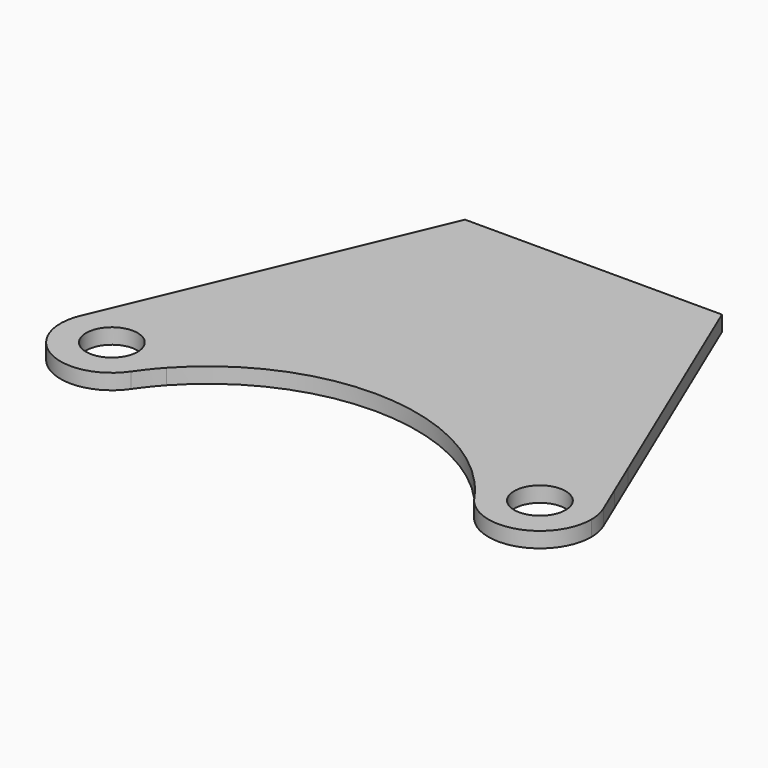
from build123d import *

# Parameters (mm, degrees)
F0_R     = 10
F1_DEPTH = 6


with BuildPart() as f1:
    # F0 (on Top) → F1 (new body)
    with BuildSketch(Plane.XY):
        with BuildLine():
            ThreePointArc((66.8107155763, 68.8983527146), (89.2220086446, 61.1485010982), (103.2801650714, 80.2454771665))
            ThreePointArc((103.2801650714, 80.2454771665), (102.8817929615, 84.2174016446), (101.7025466654, 88.0310957293))
            ThreePointArc((101.7025466654, 88.0310957293), (73.6640874011, 97.7820404055), (66.8107155763, 68.8983527146))
        make_face()
        with Locations((83.2801650714, 80.2454771665)):
            Circle(F0_R, mode=Mode.SUBTRACT)
        with BuildLine():
            ThreePointArc((66.8107155763, 68.8983527146), (73.6640874011, 97.7820404055), (101.7025466654, 88.0310957293))
            Line((101.7025466654, 88.0310957293), (96.8992238213, 99.3967496769))
            ThreePointArc((96.8992238213, 99.3967496769), (71.3236564608, 100.476441104), (59.9351524158, 77.550967172))
            ThreePointArc((59.9351524158, 77.550967172), (63.5204352748, 73.3418677958), (66.8107155763, 68.8983527146))
        make_face()
        with BuildLine():
            ThreePointArc((59.9351524158, 77.550967172), (71.3236564608, 100.476441104), (96.8992238213, 99.3967496769))
            Line((96.8992238213, 99.3967496769), (90.8352022654, 113.7454771665))
            Line((90.8352022654, 113.7454771665), (-90.8352022654, 113.7454771665))
            Line((-90.8352022654, 113.7454771665), (-96.8992238213, 99.3967496769))
            ThreePointArc((-96.8992238213, 99.3967496769), (-72.5051449003, 101.1296563534), (-59.7801650714, 80.2454771665))
            ThreePointArc((-59.7801650714, 80.2454771665), (-59.8189439032, 78.8959953041), (-59.9351524158, 77.550967172))
            ThreePointArc((-59.9351524158, 77.550967172), (0, 104), (59.9351524158, 77.550967172))
        make_face()
        with BuildLine():
            ThreePointArc((-66.8107155763, 68.8983527146), (-63.5204352748, 73.3418677958), (-59.9351524158, 77.550967172))
            ThreePointArc((-59.9351524158, 77.550967172), (-59.8189439032, 78.8959953041), (-59.7801650714, 80.2454771665))
            ThreePointArc((-59.7801650714, 80.2454771665), (-72.5051449003, 101.1296563534), (-96.8992238213, 99.3967496769))
            Line((-96.8992238213, 99.3967496769), (-101.7025466654, 88.0310957293))
            ThreePointArc((-101.7025466654, 88.0310957293), (-79.3082405933, 99.8471050565), (-63.2801650714, 80.2454771665))
            ThreePointArc((-63.2801650714, 80.2454771665), (-64.1831890032, 74.3036335933), (-66.8107155763, 68.8983527146))
        make_face()
        with BuildLine():
            ThreePointArc((-101.7025466654, 88.0310957293), (-92.8962427418, 62.7089139274), (-66.8107155763, 68.8983527146))
            ThreePointArc((-66.8107155763, 68.8983527146), (-64.1831890032, 74.3036335933), (-63.2801650714, 80.2454771665))
            ThreePointArc((-63.2801650714, 80.2454771665), (-79.3082405933, 99.8471050565), (-101.7025466654, 88.0310957293))
        make_face()
        with Locations((-83.2801650714, 80.2454771665)):
            Circle(F0_R, mode=Mode.SUBTRACT)
        Polygon((-90.8352022654, 113.7454771665), (90.8352022654, 113.7454771665), (50, 210.37), (0, 210.37), (-50, 210.37), align=None)
    extrude(amount=F1_DEPTH)


solid = f1.part
